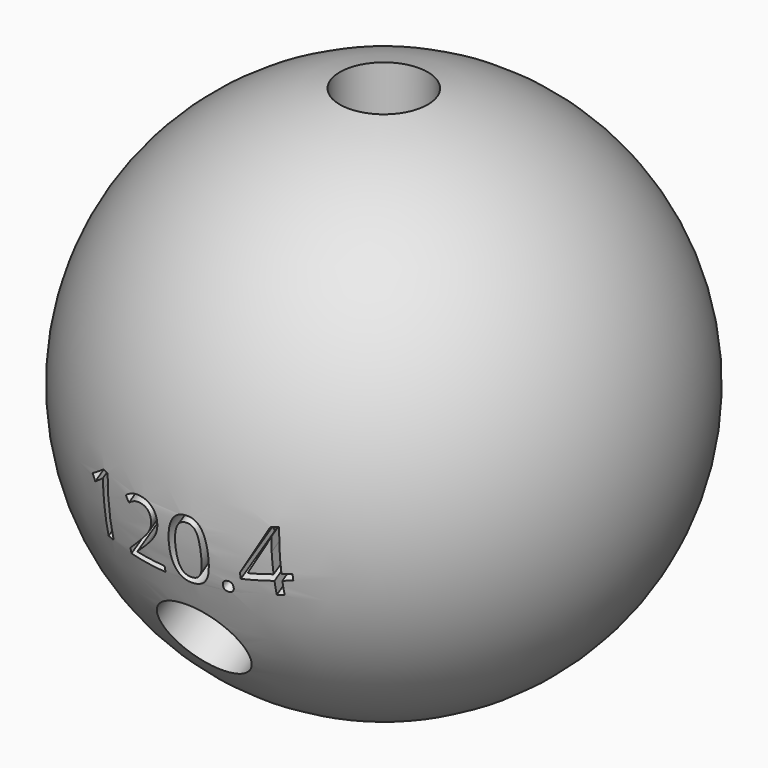
from build123d import *

# Parameters (mm, degrees)
F5_R          = 3.175
F6_DEPTH      = 76.2
F7_ANGLE      = 120.4
F8_ANGLE      = 120.9
F10_TEXT_SIZE = 5.7784387738
F11_DEPTH     = 6.35
F13_TEXT_SIZE = 6.645384969
F14_DEPTH     = 6.35


# Not quite as in the source:
# - Text() gives the source's letters only with a copy of the font that has no kerning and outlines rounded to 1/6400 em; it was checked with that copy


with BuildPart() as f2:
    # F0 (on Front) → F2 (revolve)
    with BuildSketch(Plane.XZ):
        with BuildLine():
            Line((0, -19.05), (0, 19.05))
            ThreePointArc((0, 19.05), (-19.05, 0), (0, -19.05))
        make_face()
    revolve(axis=Axis((0, 0, 0), (0, 0, 1)))

    # F10 (on offset) → F11 (cut)
    with BuildSketch(Plane(origin=(0, -17.5262777583, -10.2826060869), x_dir=(1, 0, 0), z_dir=(0, -0.8625136692, -0.5060337641))):
        with Locations((-7.3158596642, 5.1700836048)):
            Text('120.4', F10_TEXT_SIZE, font='Open Sans', text_align=(TextAlign.LEFT, TextAlign.BOTTOM))
    extrude(amount=-F11_DEPTH, mode=Mode.SUBTRACT)

    # F13 (on offset) → F14 (cut)
    with BuildSketch(Plane(origin=(0, 17.8236100465, -9.758141468), x_dir=(-1, 0, 0), z_dir=(0, 0.8771461637, -0.4802234974))):
        with Locations((-8.5071311017, 6.5649296157)):
            Text('119.5', F13_TEXT_SIZE, font='Open Sans', text_align=(TextAlign.LEFT, TextAlign.BOTTOM))
    extrude(amount=-F14_DEPTH, mode=Mode.SUBTRACT)


with BuildPart() as f6:
    # F5 (on offset) → F6 (new body)
    with BuildSketch(Plane.XY.offset(7.62)):
        Circle(F5_R)
    extrude(amount=F6_DEPTH)


with BuildPart() as f7_1:
    # F7: copy of F6
    add(f6.part.rotate(Axis((38.1614528596, 0, 0), (1, 0, 0)), F7_ANGLE))


with BuildPart() as f8_1:
    # F8: copy of F7_1
    add(f7_1.part.rotate(Axis((38.1614528596, 0, 0), (1, 0, 0)), F8_ANGLE))


with BuildPart() as f2_1:
    add(f2.part)

    # F15: cut F6, F7_1, F8_1
    add(f6.part, mode=Mode.SUBTRACT)
    add(f7_1.part, mode=Mode.SUBTRACT)
    add(f8_1.part, mode=Mode.SUBTRACT)


solid = f2_1.part
